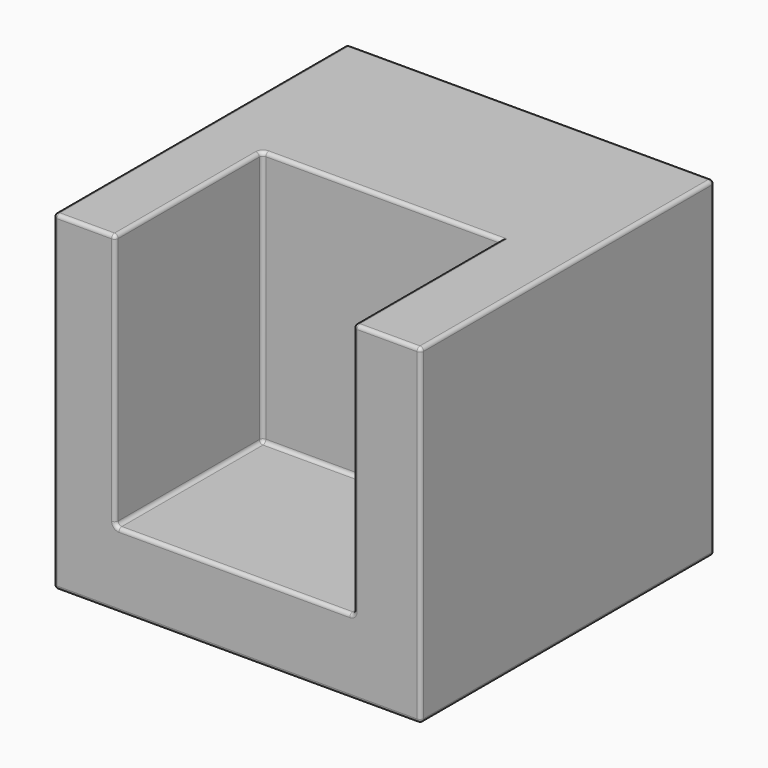
from build123d import *

# Parameters (mm, degrees)
F0_W     = 100
F0_H     = 100
F1_DEPTH = 90
F2_W     = 64.8323260248
F2_H     = 70.6382095814
F3_DEPTH = 50
F4_W     = 65.3021298349
F4_H     = 31.1890766025
F5_DEPTH = 25
F6_DEPTH = 50
F8_R     = 1


# Not quite as in the source:
# - a feature of the source that left no trace in its solid (it failed there, or was rolled back) is left out


with BuildPart() as f1:
    # F0 (on Top) → F1 (new body)
    with BuildSketch(Plane.XY):
        Rectangle(F0_W, F0_H)
    extrude(amount=F1_DEPTH)

    # F2 (on Front) → F3 (cut)
    with BuildSketch(Plane.XZ):
        with Locations((-0.7257331163, 55.6396842003)):
            Rectangle(F2_W, F2_H)
    extrude(amount=F3_DEPTH, mode=Mode.SUBTRACT)

    # F4 (on Top) → F5 (join)
    with BuildSketch(Plane.XY):
        with Locations((-0.2436619252, 15.5945383012)):
            Rectangle(F4_W, F4_H)
    extrude(amount=F5_DEPTH)

    # F4 (on Top) → F6 (join)
    with BuildSketch(Plane.XY):
        with Locations((-0.2436619252, 15.5945383012)):
            Rectangle(F4_W, F4_H)
    extrude(amount=F6_DEPTH)

    # F8
    f8_edges = [f1.edges().sort_by_distance(p)[0] for p in [
        (-33.141896, -25, 90),
        (31.69043, -25, 90),
        (40.845215, -50, 90),
        (50, 0, 90),
        (0, 50, 90),
        (-50, 0, 90),
        (-50, 50, 45),
        (-50, 0, 0),
        (-41.570948, -50, 90),
        (-33.141896, -50, 55.16029),
        (0, -50, 0),
        (-0.725733, -50, 20.320579),
        (31.69043, -25, 20.320579),
        (31.69043, -50, 55.16029),
        (50, -50, 45),
        (-0.725733, 0, 20.320579),
        (-33.141896, -25, 20.320579),
        (-33.141896, 0, 55.16029),
        (-50, -50, 45),
        (50, 50, 45),
        (50, 0, 0),
        (0, 50, 0),
        (-0.725733, 0, 90),
    ]]
    fillet(f8_edges, radius=F8_R)


solid = f1.part
